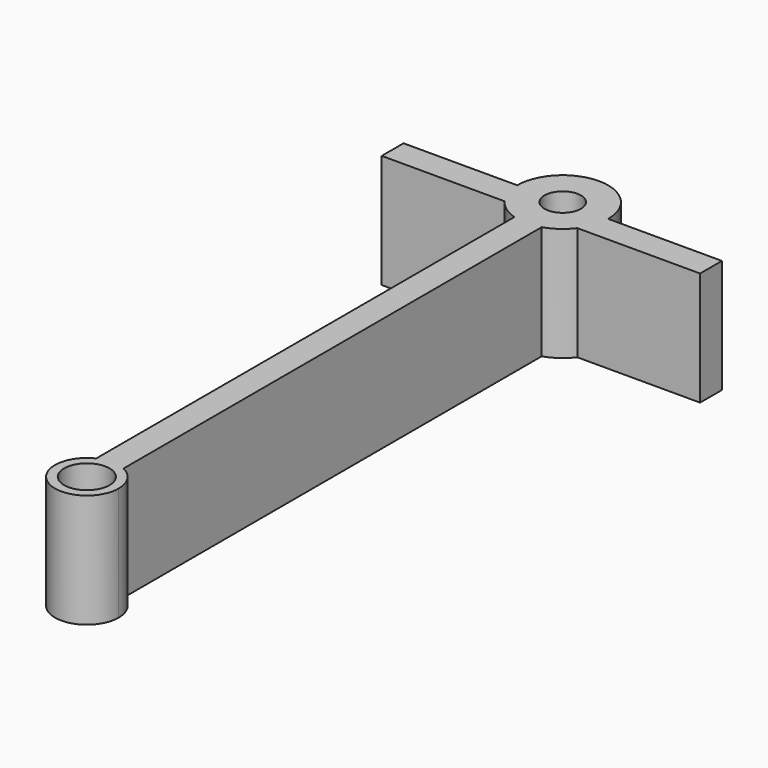
from build123d import *

# Parameters (mm, degrees)
F1_DEPTH = 25
F3_DEPTH = 25


# Not quite as in the source:
# - a feature names something its author has since deleted; it is built from what else it names


with BuildPart() as f1:
    # F0 (on Top) → F1 (new body)
    with BuildSketch(Plane.XY):
        with BuildLine():
            Line((-3, -126.7858377695), (-3, -124.4612824492))
            ThreePointArc((-3, -124.4612824492), (-3.7416573868, -136.7019175526), (7, -130.7858377695))
            ThreePointArc((7, -130.7858377695), (5.9160797831, -127.0441803827), (3, -124.4612824492))
            Line((3, -124.4612824492), (3, -126.7858377695))
            ThreePointArc((3, -126.7858377695), (4.472135955, -128.549769792), (5, -130.7858377695))
            ThreePointArc((5, -130.7858377695), (-2.2360679775, -135.2579737245), (-3, -126.7858377695))
        make_face()
        with BuildLine():
            ThreePointArc((3, -9.5393920142), (0, -10), (-3, -9.5393920142))
            Line((-3, -9.5393920142), (-3, -124.4612824492))
            ThreePointArc((-3, -124.4612824492), (0, -123.7858377695), (3, -124.4612824492))
            Line((3, -124.4612824492), (3, -9.5393920142))
        make_face()
        with BuildLine():
            ThreePointArc((3, -124.4612824492), (0, -123.7858377695), (-3, -124.4612824492))
            Line((-3, -124.4612824492), (-3, -126.7858377695))
            ThreePointArc((-3, -126.7858377695), (0, -125.7858377695), (3, -126.7858377695))
            Line((3, -126.7858377695), (3, -124.4612824492))
        make_face()
        with BuildLine():
            ThreePointArc((-3, -2.6457513111), (-1.4142135624, 3.7416573868), (4, 0))
            ThreePointArc((4, 0), (3.7416573868, -1.4142135624), (3, -2.6457513111))
            Line((3, -2.6457513111), (3, -9.5393920142))
            ThreePointArc((3, -9.5393920142), (8.0622577483, -5.9160797831), (10, 0))
            ThreePointArc((10, 0), (-5.9160797831, 8.0622577483), (-3, -9.5393920142))
            Line((-3, -9.5393920142), (-3, -2.6457513111))
        make_face()
        with BuildLine():
            ThreePointArc((3, -2.6457513111), (0, -4), (-3, -2.6457513111))
            Line((-3, -2.6457513111), (-3, -9.5393920142))
            ThreePointArc((-3, -9.5393920142), (0, -10), (3, -9.5393920142))
            Line((3, -9.5393920142), (3, -2.6457513111))
        make_face()
    extrude(amount=F1_DEPTH)

    # F2 (on Top) → F3 (join)
    with BuildSketch(Plane.XY):
        with BuildLine():
            Line((35, 0), (4, 0))
            ThreePointArc((4, 0), (0, -4), (-4, 0))
            Line((-4, 0), (-35, 0))
            Line((-35, 0), (-35, -6))
            Line((-35, -6), (35, -6))
            Line((35, -6), (35, 0))
        make_face()
    extrude(amount=F3_DEPTH)


solid = f1.part
